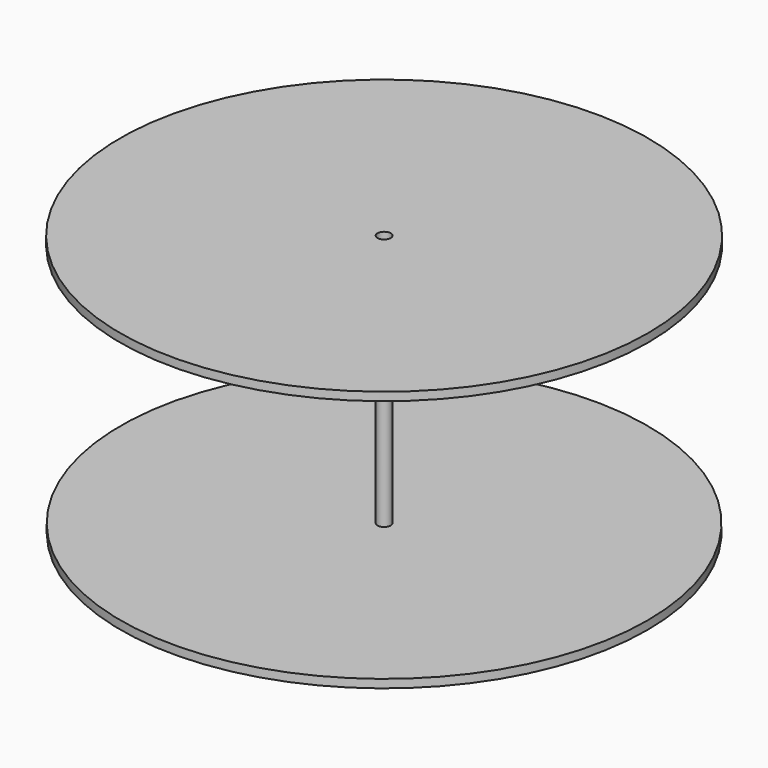
from build123d import *

# Parameters (mm, degrees)
F0_R     = 200
F1_DEPTH = 6.35
F2_R     = 5
F3_DEPTH = 185.7502
F4_R     = 200.3737721093
F4_R_2   = 5
F5_DEPTH = 6.35


# Not quite as in the source:
# - a length typed as a fraction of an inch, garbled in the dataset ("3 / 203.2 mm" for 3/8 in), is restored


with BuildPart() as f1:
    # F0 (on Top) → F1 (new body)
    with BuildSketch(Plane.XY):
        Circle(F0_R)
    extrude(amount=F1_DEPTH)

    # F2 (on face) → F3 (join)
    with BuildSketch(Plane.XY.offset(6.35)):
        Circle(F2_R)
    extrude(amount=F3_DEPTH)


with BuildPart() as f5:
    # F4 (on face) → F5 (new body)
    with BuildSketch(Plane.XY.offset(192.1002)):
        Circle(F4_R)
        Circle(F4_R_2, mode=Mode.SUBTRACT)
    extrude(amount=F5_DEPTH)


solid = Compound([f1.part, f5.part])
